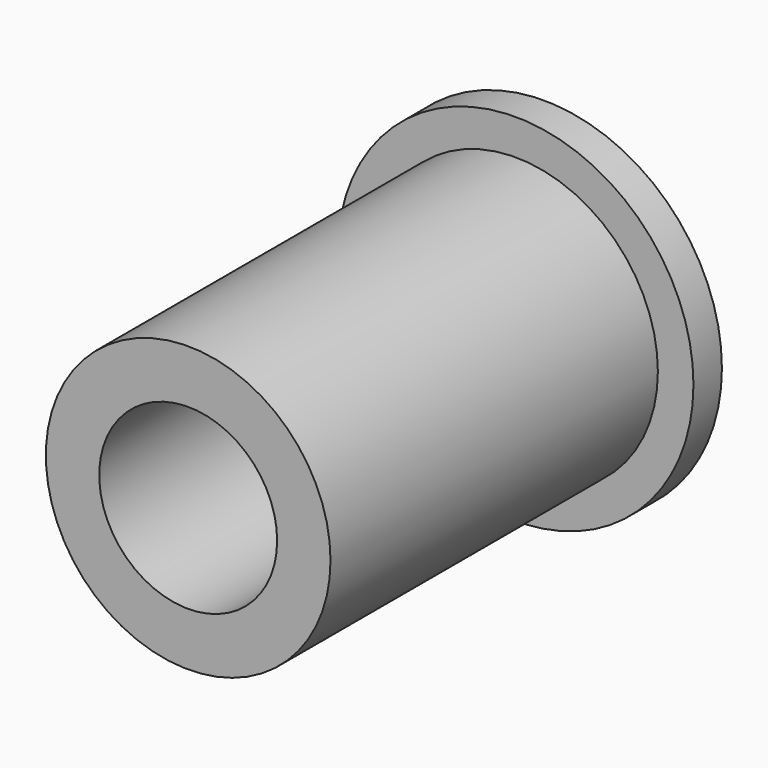
from build123d import *

# Parameters (mm, degrees)
F0_R     = 8
F0_R_2   = 5
F1_DEPTH = 11.5
F2_R     = 10
F2_R_2   = 8
F2_R_3   = 5
F3_DEPTH = 2


with BuildPart() as f1:
    # F0 (on Front) → F1 (new body, symmetric)
    with BuildSketch(Plane.XZ):
        Circle(F0_R)
        Circle(F0_R_2, mode=Mode.SUBTRACT)
    extrude(amount=F1_DEPTH, both=True)

    # F2 (on face) → F3 (join)
    with BuildSketch(Plane(origin=(0, 11.5, 0), x_dir=(-1, 0, 0), z_dir=(0, 1, 0))):
        Circle(F2_R)
        Circle(F2_R_2, mode=Mode.SUBTRACT)
        Circle(F2_R_2)
        Circle(F2_R_3, mode=Mode.SUBTRACT)
    extrude(amount=F3_DEPTH)


solid = f1.part
